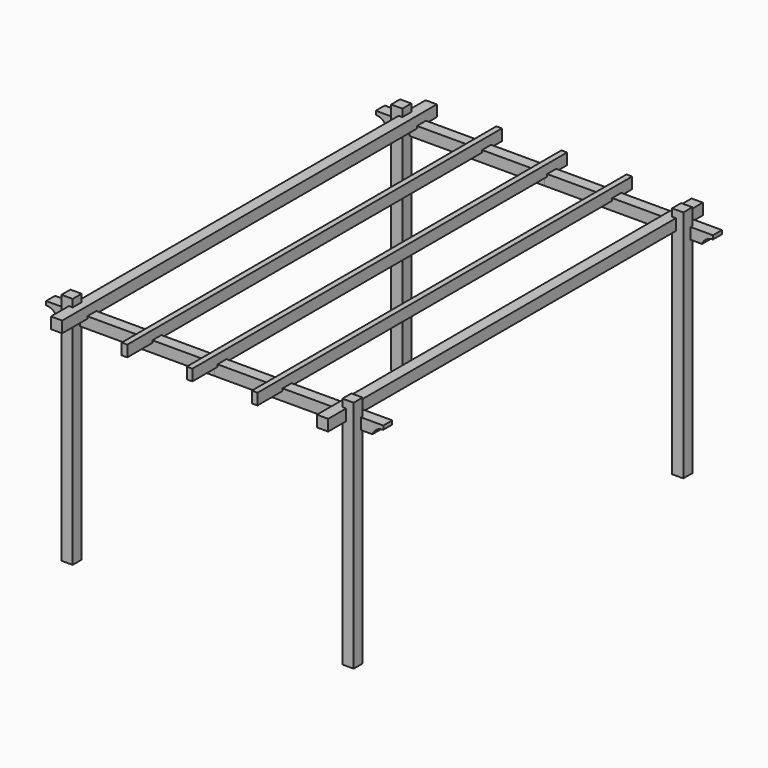
from build123d import *

# Parameters (mm, degrees)
F1_W           = 120
F1_H           = 120
F2_DEPTH       = 2500
F5_W           = 120
F5_H           = 120
F6_DEPTH       = 2500
F7_DEPTH       = 2500
F8_W           = 60
F8_H           = 120
F9_DEPTH       = 2500
F10_W          = 120
F10_H          = 120
F11_DEPTH      = 1800
F12_DEPTH      = 1800.001
F14_R          = 125
F15_DEPTH      = 2500.001
F15_DEPTH_BACK = 2500.001


with BuildPart() as f2:
    # F1 (on Top) → F2 (new body)
    with BuildSketch(Plane.XY):
        with Locations((-1500, -2200)):
            Rectangle(F1_W, F1_H)
    extrude(amount=F2_DEPTH)


with BuildPart() as f3_1:
    # F3: instance of F2
    add(f2.part.mirror(Plane.XZ))


with BuildPart() as f4_1:
    # F4: instance of F2
    add(f2.part.mirror(Plane.YZ))


with BuildPart() as f4_2:
    # F4: instance of F3_1
    add(f3_1.part.mirror(Plane.YZ))


with BuildPart() as f6:
    # F5 (on Front) → F6 (new body, symmetric)
    with BuildSketch(Plane.XZ):
        with Locations((-1420, 2360)):
            Rectangle(F5_W, F5_H)
    extrude(amount=F6_DEPTH, both=True)


with BuildPart() as f7_tool:
    # F5 (on Front) → F7 (new body, symmetric)
    with BuildSketch(Plane.XZ):
        with Locations((-1420, 2360)):
            Rectangle(F5_W, F5_H)
    extrude(amount=F7_DEPTH, both=True)


with BuildPart() as f2_1:
    add(f2.part)

    # F7: cut by f7_tool
    add(f7_tool.part, mode=Mode.SUBTRACT)


with BuildPart() as f3_1_1:
    add(f3_1.part)

    # F7: cut by f7_tool
    add(f7_tool.part, mode=Mode.SUBTRACT)


with BuildPart() as f9:
    # F8 (on Front) → F9 (new body, symmetric)
    with BuildSketch(Plane.XZ):
        with Locations((0, 2360)):
            Rectangle(F8_W, F8_H)
    extrude(amount=F9_DEPTH, both=True)


with BuildPart() as f9b:
    # F8 (on Front) → F9, piece 2 (new body, symmetric)
    with BuildSketch(Plane.XZ):
        with Locations((-695, 2360)):
            Rectangle(F8_W, F8_H)
    extrude(amount=F9_DEPTH, both=True)


with BuildPart() as f11:
    # F10 (on Right) → F11 (new body)
    with BuildSketch(Plane.YZ):
        with Locations((2295, 2265)):
            Rectangle(F10_W, F10_H)
    extrude(amount=-F11_DEPTH)


with BuildPart() as f11b:
    # F10 (on Right) → F11, piece 2 (new body)
    with BuildSketch(Plane.YZ):
        with Locations((-2105, 2265)):
            Rectangle(F10_W, F10_H)
    extrude(amount=-F11_DEPTH)


with BuildPart() as f12_tool:
    # F10 (on Right) → F12 (new body, through all)
    with BuildSketch(Plane.YZ):
        with Locations((2295, 2265)):
            Rectangle(F10_W, F10_H)
        with Locations((-2105, 2265)):
            Rectangle(F10_W, F10_H)
    extrude(amount=-F12_DEPTH)


with BuildPart() as f2_2:
    add(f2_1.part)

    # F12: cut by f12_tool
    add(f12_tool.part, mode=Mode.SUBTRACT)


with BuildPart() as f3_1_2:
    add(f3_1_1.part)

    # F12: cut by f12_tool
    add(f12_tool.part, mode=Mode.SUBTRACT)


with BuildPart() as f6_1:
    add(f6.part)

    # F12: cut by f12_tool
    add(f12_tool.part, mode=Mode.SUBTRACT)


with BuildPart() as f9_1:
    add(f9.part)

    # F12: cut by f12_tool
    add(f12_tool.part, mode=Mode.SUBTRACT)


with BuildPart() as f9b_1:
    add(f9b.part)

    # F12: cut by f12_tool
    add(f12_tool.part, mode=Mode.SUBTRACT)


with BuildPart() as f13_1:
    # F13: instance of F9b
    add(f9b_1.part.mirror(Plane.YZ))


with BuildPart() as f13_2:
    # F13: instance of F6
    add(f6_1.part.mirror(Plane.YZ))


with BuildPart() as f13_3:
    # F13: instance of F11
    add(f11.part.mirror(Plane.YZ))


with BuildPart() as f13_4:
    # F13: instance of F11b
    add(f11b.part.mirror(Plane.YZ))


with BuildPart() as f13_5:
    # F13: instance of F2
    add(f2_2.part.mirror(Plane.YZ))


with BuildPart() as f13_6:
    # F13: instance of F3_1
    add(f3_1_2.part.mirror(Plane.YZ))


with BuildPart() as f15_tool:
    # F14 (on Front) → F15 (new body, two sides)
    with BuildSketch(Plane.XZ) as f15_sk:
        with Locations((1800, 2160)):
            Circle(F14_R)
        with Locations((-1800, 2160)):
            Circle(F14_R)
    extrude(amount=F15_DEPTH)
    extrude(f15_sk.sketch, amount=-F15_DEPTH_BACK)


with BuildPart() as f11_1:
    add(f11.part)

    # F15: cut by f15_tool
    add(f15_tool.part, mode=Mode.SUBTRACT)


with BuildPart() as f11b_1:
    add(f11b.part)

    # F15: cut by f15_tool
    add(f15_tool.part, mode=Mode.SUBTRACT)


with BuildPart() as f13_3_1:
    add(f13_3.part)

    # F15: cut by f15_tool
    add(f15_tool.part, mode=Mode.SUBTRACT)


with BuildPart() as f13_4_1:
    add(f13_4.part)

    # F15: cut by f15_tool
    add(f15_tool.part, mode=Mode.SUBTRACT)


solid = Compound([f4_1.part, f4_2.part, f2_2.part, f3_1_2.part, f6_1.part, f9_1.part, f9b_1.part, f13_1.part, f13_2.part, f13_5.part, f13_6.part, f11_1.part, f11b_1.part, f13_3_1.part, f13_4_1.part])
